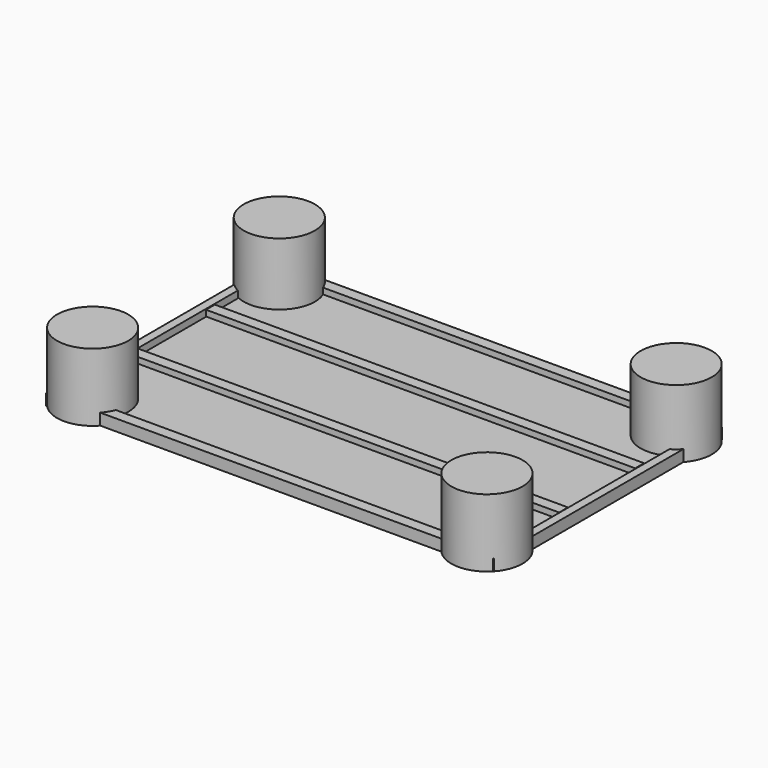
from build123d import *

# Parameters (mm, degrees)
F0_W      = 6.0556903481
F0_H      = 132.6194964349
F1_DEPTH  = 2.54
F2_W      = 200.3036439419
F2_H      = 5.1624625921
F4_DEPTH  = 5.334
F5_DEPTH  = 5.334
F6_DEPTH  = 5.334
F7_W      = 3.9294064045
F7_H      = 133.2067586482
F8_DEPTH  = 5.334
F9_R      = 16.621019502
F10_DEPTH = 31.75


# Not quite as in the source:
# - the program builds the solid bodies; features that only make, move or delete a surface that nothing else refers to are left out


with BuildPart() as f1:
    # F0 (on Top) → F1 (new body)
    with BuildSketch(Plane.XY):
        with Locations((-97.3073802888, 10.3850681335)):
            Rectangle(F0_W, F0_H)
        with Locations((-91.2516899407, 10.3850681335)):
            Rectangle(F0_W, F0_H)
        with Locations((-85.1959995925, 10.3850681335)):
            Rectangle(F0_W, F0_H)
        with Locations((-79.1403092444, 10.3850681335)):
            Rectangle(F0_W, F0_H)
        with Locations((-73.0846188962, 10.3850681335)):
            Rectangle(F0_W, F0_H)
        with Locations((-67.0289285481, 10.3850681335)):
            Rectangle(F0_W, F0_H)
        with Locations((-60.9732381999, 10.3850681335)):
            Rectangle(F0_W, F0_H)
        with Locations((-54.9175478518, 10.3850681335)):
            Rectangle(F0_W, F0_H)
        with Locations((-48.8618575037, 10.3850681335)):
            Rectangle(F0_W, F0_H)
        with Locations((-42.8061671555, 10.3850681335)):
            Rectangle(F0_W, F0_H)
        with Locations((-36.7504768074, 10.3850681335)):
            Rectangle(F0_W, F0_H)
        with Locations((-30.6947864592, 10.3850681335)):
            Rectangle(F0_W, F0_H)
        with Locations((-24.6390961111, 10.3850681335)):
            Rectangle(F0_W, F0_H)
        with Locations((-18.5834057629, 10.3850681335)):
            Rectangle(F0_W, F0_H)
        with Locations((-12.5277154148, 10.3850681335)):
            Rectangle(F0_W, F0_H)
        with Locations((-6.4720250666, 10.3850681335)):
            Rectangle(F0_W, F0_H)
        with Locations((-0.4163347185, 10.3850681335)):
            Rectangle(F0_W, F0_H)
        with Locations((5.6393556297, 10.3850681335)):
            Rectangle(F0_W, F0_H)
        with Locations((11.6950459778, 10.3850681335)):
            Rectangle(F0_W, F0_H)
        with Locations((17.750736326, 10.3850681335)):
            Rectangle(F0_W, F0_H)
        with Locations((23.8064266741, 10.3850681335)):
            Rectangle(F0_W, F0_H)
        with Locations((29.8621170223, 10.3850681335)):
            Rectangle(F0_W, F0_H)
        with Locations((35.9178073704, 10.3850681335)):
            Rectangle(F0_W, F0_H)
        with Locations((41.9734977186, 10.3850681335)):
            Rectangle(F0_W, F0_H)
        with Locations((48.0291880667, 10.3850681335)):
            Rectangle(F0_W, F0_H)
        with Locations((54.0848784149, 10.3850681335)):
            Rectangle(F0_W, F0_H)
        with Locations((60.140568763, 10.3850681335)):
            Rectangle(F0_W, F0_H)
        with Locations((66.1962591112, 10.3850681335)):
            Rectangle(F0_W, F0_H)
        with Locations((72.2519494593, 10.3850681335)):
            Rectangle(F0_W, F0_H)
        with Locations((78.3076398075, 10.3850681335)):
            Rectangle(F0_W, F0_H)
        with Locations((84.3633301556, 10.3850681335)):
            Rectangle(F0_W, F0_H)
        with Locations((90.4190205038, 10.3850681335)):
            Rectangle(F0_W, F0_H)
        with Locations((96.4747108519, 10.3850681335)):
            Rectangle(F0_W, F0_H)
    extrude(amount=F1_DEPTH)

    # F2 (on Top) → F4 (join)
    with BuildSketch(Plane.XY):
        with Locations((-0.2800673246, 34.1405831277)):
            Rectangle(F2_W, F2_H)
    extrude(amount=F4_DEPTH)

    # F2 (on Top) → F5 (join)
    with BuildSketch(Plane.XY):
        with Locations((-0.1398418099, -10.4263699614)):
            Rectangle(F2_W, F2_H)
    extrude(amount=F5_DEPTH)

    # F2 (on Top) → F6 (join)
    with BuildSketch(Plane.XY):
        with Locations((-0.5909577012, 74.434235692)):
            Rectangle(F2_W, F2_H)
        with Locations((-0.2800673246, 34.1405831277)):
            Rectangle(F2_W, F2_H)
        with Locations((-0.2306103706, -53.3664822578)):
            Rectangle(F2_W, F2_H)
        with Locations((-0.1398418099, -10.4263699614)):
            Rectangle(F2_W, F2_H)
    extrude(amount=F6_DEPTH)


with BuildPart() as f8:
    # F7 (on Top) → F8 (new body)
    with BuildSketch(Plane.XY):
        with Locations((102.1542623639, 10.2424006909)):
            Rectangle(F7_W, F7_H)
    extrude(amount=F8_DEPTH)


with BuildPart() as f8b:
    # F7 (on Top) → F8, piece 2 (new body)
    with BuildSketch(Plane.XY):
        with Locations((-102.8498336673, 10.3216152638)):
            Rectangle(F7_W, F7_H)
    extrude(amount=F8_DEPTH)


with BuildPart() as f10:
    # F9 (on Top) → F10 (new body)
    with BuildSketch(Plane.XY):
        with Locations((91.8380022049, 65.513715148)):
            Circle(F9_R)
    extrude(amount=F10_DEPTH)


with BuildPart() as f10b:
    # F9 (on Top) → F10, piece 2 (new body)
    with BuildSketch(Plane.XY):
        with Locations((91.8380022049, -44.8967292905)):
            Circle(F9_R)
    extrude(amount=F10_DEPTH)


with BuildPart() as f10c:
    # F9 (on Top) → F10, piece 3 (new body)
    with BuildSketch(Plane.XY):
        with Locations((-93.3917686343, 65.513715148)):
            Circle(F9_R)
    extrude(amount=F10_DEPTH)


with BuildPart() as f10d:
    # F9 (on Top) → F10, piece 4 (new body)
    with BuildSketch(Plane.XY):
        with Locations((-92.2020450234, -44.8967292905)):
            Circle(F9_R)
    extrude(amount=F10_DEPTH)


solid = Compound([f1.part, f8.part, f8b.part, f10.part, f10b.part, f10c.part, f10d.part])
